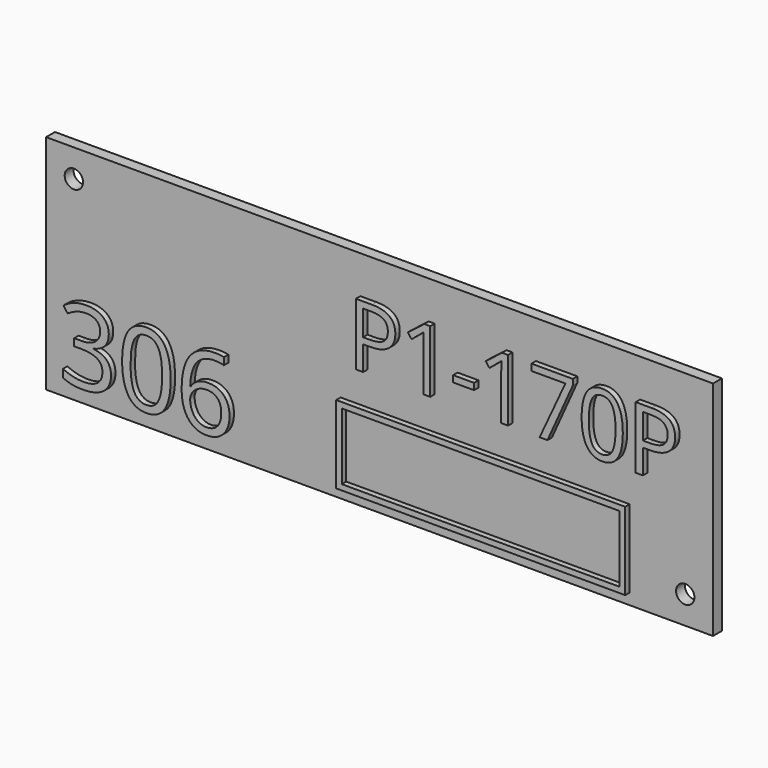
from build123d import *

# Parameters (mm, degrees)
F0_W         = 120
F0_H         = 40
F1_DEPTH     = 2
F3_D         = 3.3
F4_TEXT_SIZE = 15.681149951
F5_DEPTH     = 1
F6_TEXT_SIZE = 18.4837545126
F7_DEPTH     = 1
F8_W         = 52
F8_H         = 14
F8_W_2       = 49.99999962
F8_H_2       = 11.99999962
F9_DEPTH     = 1


# Not quite as in the source:
# - Text() gives the source's letters only with a copy of the font that has no kerning and outlines rounded to 1/6400 em; it was checked with that copy


with BuildPart() as f1:
    # F0 (on Front) → F1 (new body)
    with BuildSketch(Plane.XZ):
        Rectangle(F0_W, F0_H)
    extrude(amount=F1_DEPTH)

    # F3 (through all)
    with Locations(Plane.XZ.offset(2)):
        with Locations((-55, 15), (55, -15)):
            Hole(F3_D / 2)

    # F4 (on face) → F5 (join)
    with BuildSketch(Plane.XZ.offset(2)):
        with Locations((-5, 2)):
            Text('P1-170P', F4_TEXT_SIZE, font='Open Sans', text_align=(TextAlign.LEFT, TextAlign.BOTTOM))
    extrude(amount=F5_DEPTH)

    # F6 (on face) → F7 (join)
    with BuildSketch(Plane.XZ.offset(2)):
        with Locations((-57, -17)):
            Text('306', F6_TEXT_SIZE, font='Open Sans', text_align=(TextAlign.LEFT, TextAlign.BOTTOM))
    extrude(amount=F7_DEPTH)

    # F8 (on face) → F9 (join)
    with BuildSketch(Plane.XZ.offset(2)):
        with Locations((19, -11)):
            Rectangle(F8_W, F8_H)
        with Locations((19, -11)):
            Rectangle(F8_W_2, F8_H_2, mode=Mode.SUBTRACT)
    extrude(amount=F9_DEPTH)


solid = f1.part
